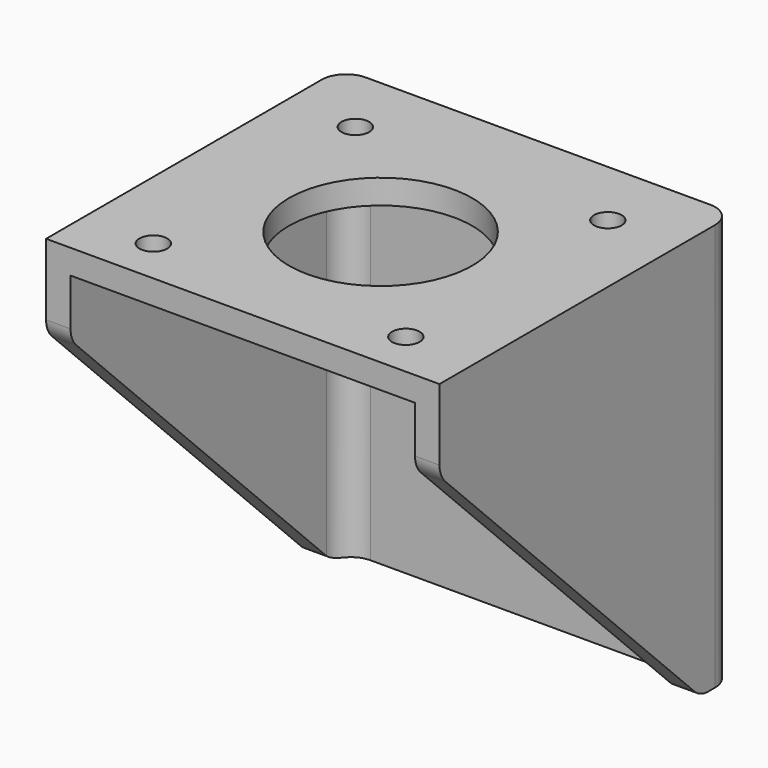
from build123d import *

# Parameters (mm, degrees)
F1_W     = 42.3
F1_H     = 42.3
F1_R     = 1.625
F2_DEPTH = 50
F4_T     = -3
F5_D     = 3.4
F6_D     = 6.6
F7_D     = 22.5
F8_SIZE  = 40
F9_R     = 3


with BuildPart() as f2:
    # F1 (on Top) → F2 (new body)
    with BuildSketch(Plane.XY):
        Rectangle(F1_W, F1_H)
        with Locations((-15.5, -15.5)):
            Circle(F1_R, mode=Mode.SUBTRACT)
        with Locations((15.5, -15.5)):
            Circle(F1_R, mode=Mode.SUBTRACT)
        with Locations((-15.5, 15.5)):
            Circle(F1_R, mode=Mode.SUBTRACT)
        with Locations((15.5, 15.5)):
            Circle(F1_R, mode=Mode.SUBTRACT)
        with Locations((-15.5, 15.5)):
            Circle(F1_R)
        with Locations((15.5, 15.5)):
            Circle(F1_R)
        with Locations((-15.5, -15.5)):
            Circle(F1_R)
        with Locations((15.5, -15.5)):
            Circle(F1_R)
        Polygon((-21.15, 21.15), (21.15, 21.15), (21.15, -21.15), (24.15, -21.15), (24.15, 24.15), (-24.15, 24.15), (-24.15, -21.15), (-21.15, -21.15), align=None)
    extrude(amount=F2_DEPTH)

    # F4
    f4_openings = [f2.faces().sort_by_distance(p)[0] for p in [
        (0, -21.15, 25),
        (0, 1.5, 0),
    ]]
    offset(amount=F4_T, openings=f4_openings)

    # F5 (through all)
    with Locations(Plane(origin=(0, 0, 0), x_dir=(1, 0, 0), z_dir=(0, 0, -1))):
        with Locations((-15.5, 15.5), (15.5, 15.5), (15.5, -15.5), (-15.5, -15.5)):
            Hole(F5_D / 2)

    # F6 (through all)
    with Locations(Plane.XZ.offset(21.15)):
        with Locations((0, 33.5), (0, 13.5)):
            Hole(F6_D / 2)

    # F7 (through all)
    with Locations(Plane(origin=(0, 0, 0), x_dir=(1, 0, 0), z_dir=(0, 0, -1))):
        with Locations((0, 0)):
            Hole(F7_D / 2)

    # F8
    f8_edges = [f2.edges().sort_by_distance(p)[0] for p in [
        (-22.65, -21.15, 0),
        (22.65, -21.15, 0),
    ]]
    chamfer(f8_edges, length=F8_SIZE)

    # F9 (call 1 of 8: OpenCascade refuses the feature's edges together)
    f9_edges = [f2.edges().sort_by_distance(p)[0] for p in [
        (-22.65, -21.15, 40),
    ]]
    fillet(f9_edges, radius=F9_R)

    # F9#2 (call 2 of 8)
    f9_2_edges = [f2.edges().sort_by_distance(p)[0] for p in [
        (22.65, -21.15, 40),
    ]]
    fillet(f9_2_edges, radius=F9_R)

    # F9#3 (call 3 of 8)
    f9_3_edges = [f2.edges().sort_by_distance(p)[0] for p in [
        (-22.65, 18.85, 0),
    ]]
    fillet(f9_3_edges, radius=F9_R)

    # F9#4 (call 4 of 8)
    f9_4_edges = [f2.edges().sort_by_distance(p)[0] for p in [
        (22.65, 18.85, 0),
    ]]
    fillet(f9_4_edges, radius=F9_R)

    # F9#5 (call 5 of 8)
    f9_5_edges = [f2.edges().sort_by_distance(p)[0] for p in [
        (-21.15, 21.15, 23.5),
    ]]
    fillet(f9_5_edges, radius=F9_R)

    # F9#6 (call 6 of 8)
    f9_6_edges = [f2.edges().sort_by_distance(p)[0] for p in [
        (21.15, 21.15, 23.5),
    ]]
    fillet(f9_6_edges, radius=F9_R)

    # F9#7 (call 7 of 8)
    f9_7_edges = [f2.edges().sort_by_distance(p)[0] for p in [
        (-24.15, 24.15, 25),
    ]]
    fillet(f9_7_edges, radius=F9_R)

    # F9#8 (call 8 of 8)
    f9_8_edges = [f2.edges().sort_by_distance(p)[0] for p in [
        (24.15, 24.15, 25),
    ]]
    fillet(f9_8_edges, radius=F9_R)


solid = f2.part
